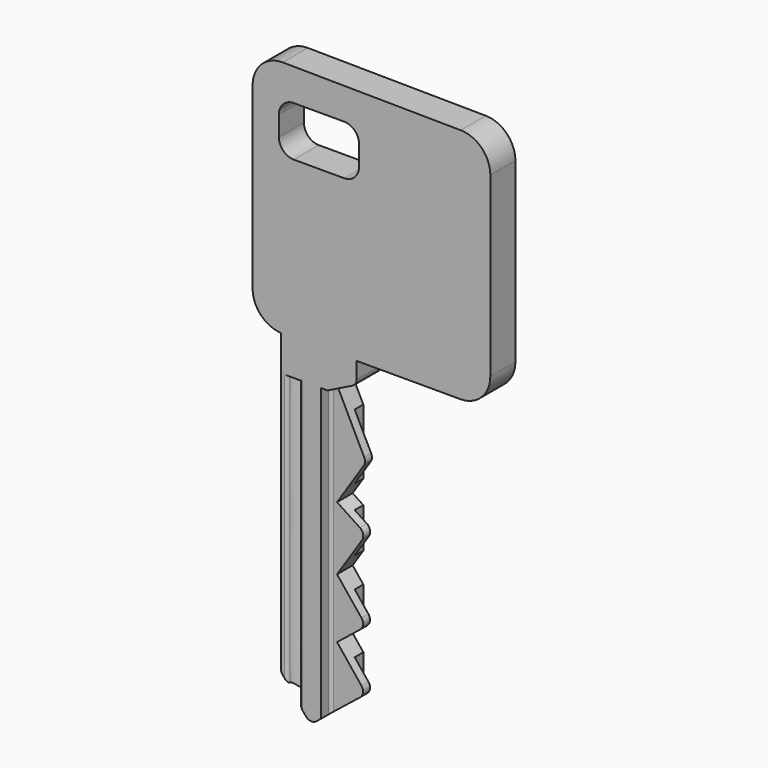
from build123d import *

# Parameters (mm, degrees)
F0_W        = 13.6487651616
F0_H        = 8.4716491401
F1_DEPTH    = 5.334
F2_T1_DEPTH = 30.734
F2_T3_DEPTH = 30.9986733357
F2_T5_DEPTH = 30.6972722749
F2_T7_DEPTH = 30.472056174
F3_R        = 2.54
F4_R        = 1.27
F6_DEPTH    = 52.1462
F7_W        = 6.471471861
F7_H        = 2.0470987074
F8_DEPTH    = 58.928
F9_W        = 3.0602971092
F9_H        = 1.8379887333
F10_DEPTH   = 54.61
F12_DEPTH   = 55.626
F13_R       = 0.508


# Not quite as in the source:
# - a fillet or chamfer that OpenCascade refuses, or shapes differently, is made with other operations: its cross-section is extruded or revolved along the edge and cut away or added


with BuildPart() as f1:
    # F0 (on Front) → F1 (new body)
    with BuildSketch(Plane.XZ):
        Polygon((40.4473207891, 46.2965518236), (0, 46.7158481479), (0, 6.0438592918), (4.8069125041, 6.0438592918), (4.8069125041, -44.6913056076), (9.8384991288, -50.9807877243), (17.7003503195, -44.6913056076), (12.7505768579, -38.5040899258), (17.7003503195, -34.5442704236), (12.7505768579, -28.3570547418), (17.7003503195, -20.7912679762), (12.7505768579, -17.5529719363), (17.7003503195, -9.9871851707), (12.7505768579, 0), (17.7003503195, 2.4531694269), (17.7003503195, 6.0438592918), (40.4473207891, 6.0438592918), align=None)
        with Locations((11.2955300137, 36.9457956403)):
            Rectangle(F0_W, F0_H, mode=Mode.SUBTRACT)
    extrude(amount=F1_DEPTH)

    # F2: fillet of radius 5.08 on 4 edges, made by hand

    # F2_s2 → F2_t1 (cut)
    with BuildSketch(Plane.XZ.offset(-12.7)):
        with BuildLine():
            ThreePointArc((35.3673207891, 6.0438592918), (38.9594232375, 7.5317568434), (40.4473207891, 11.1238592918))
            Line((40.4473207891, 11.1238592918), (40.4473207891, 6.0438592918))
            Line((40.4473207891, 6.0438592918), (35.3673207891, 6.0438592918))
        make_face()
    extrude(amount=F2_T1_DEPTH, mode=Mode.SUBTRACT)

    # F2_s4 → F2_t3 (cut)
    with BuildSketch(Plane.XZ.offset(-12.8323366678)):
        with BuildLine():
            ThreePointArc((5.1326588868, 46.6626405444), (1.5065637787, 45.1935856581), (0, 41.5829134807))
            Line((0, 41.5829134807), (0, 46.7158481479))
            Line((0, 46.7158481479), (5.1326588868, 46.6626405444))
        make_face()
    extrude(amount=F2_T3_DEPTH, mode=Mode.SUBTRACT)

    # F2_s6 → F2_t5 (cut)
    with BuildSketch(Plane.XZ.offset(-12.6816361374)):
        with BuildLine():
            ThreePointArc((0, 11.1165137468), (1.392610376, 7.6222959859), (4.8069125041, 6.0438592918))
            Line((4.8069125041, 6.0438592918), (0, 6.0438592918))
            Line((0, 6.0438592918), (0, 11.1165137468))
        make_face()
    extrude(amount=F2_T5_DEPTH, mode=Mode.SUBTRACT)

    # F2_s8 → F2_t7 (cut)
    with BuildSketch(Plane.XZ.offset(-12.569028087)):
        with BuildLine():
            ThreePointArc((40.4473207891, 41.2689405888), (38.9779929665, 44.8423768101), (35.4199796759, 46.3486676525))
            Line((35.4199796759, 46.3486676525), (40.4473207891, 46.2965518236))
            Line((40.4473207891, 46.2965518236), (40.4473207891, 41.2689405888))
        make_face()
    extrude(amount=F2_T7_DEPTH, mode=Mode.SUBTRACT)

    # F3
    f3_edges = [f1.edges().sort_by_distance(p)[0] for p in [
        (18.119913, -2.667, 41.18162),
        (4.471147, -2.667, 41.18162),
        (4.471147, -2.667, 32.709971),
        (18.119913, -2.667, 32.709971),
    ]]
    fillet(f3_edges, radius=F3_R)

    # F4
    f4_edges = [f1.edges().sort_by_distance(p)[0] for p in [
        (17.70035, -2.667, 2.453169),
        (17.70035, -2.667, -9.987185),
        (17.70035, -2.667, -20.791268),
        (17.70035, -2.667, -34.54427),
        (17.70035, -2.667, -44.691306),
        (9.838499, -2.667, -50.980788),
        (4.806913, -2.667, -44.691306),
    ]]
    fillet(f4_edges, radius=F4_R)

    # F5 (on Top) → F6 (cut)
    with BuildSketch(Plane.XY):
        with BuildLine():
            add(Edge.make_bspline(
                [(5.9925829992, -5.3615476936), (5.9662371728, -5.1413136829), (5.9117415486, -4.685765632), (6.3531394911, -4.0979348233), (6.8182620743, -3.382318142), (7.2587507478, -3.2452825018), (7.6600250696, -4.1522550659), (8.0135536671, -4.7405594262), (8.0147180391, -5.162214979), (8.0152684823, -5.3615476936)],
                knots=[0, 0, 0, 0, 0.1405767765, 0.2907792323, 0.4524560789, 0.5501663785, 0.7152294594, 0.8653780686, 1, 1, 1, 1], degree=3))
            Line((5.9925829992, -5.3615476936), (8.0152684823, -5.3615476936))
        make_face()
    extrude(amount=-F6_DEPTH, mode=Mode.SUBTRACT)

    # F7 (on Top) → F8 (cut)
    with BuildSketch(Plane.XY):
        with Locations((14.903399162, -4.3372439686)):
            Rectangle(F7_W, F7_H)
    extrude(amount=-F8_DEPTH, mode=Mode.SUBTRACT)

    # F9 (on Top) → F10 (cut)
    with BuildSketch(Plane.XY):
        with Locations((16.1025538109, -0.9189943667)):
            Rectangle(F9_W, F9_H)
    extrude(amount=-F10_DEPTH, mode=Mode.SUBTRACT)

    # F11 (on Top) → F12 (cut)
    with BuildSketch(Plane.XY):
        with BuildLine():
            add(Edge.make_bspline(
                [(11.2238610163, 0), (11.2478981656, -0.3069122797), (11.3009665063, -0.984502007), (10.6443157535, -2.3913685017), (9.025430434, -2.589119864), (8.3644189358, -0.856075456), (8.4617577104, -0.2545179476), (8.5029415786, 0)],
                knots=[0, 0, 0, 0, 0.1796332137, 0.3965876516, 0.6003917954, 0.8309264556, 1, 1, 1, 1], degree=3))
            Line((11.2238610163, 0), (8.5029415786, 0))
        make_face()
    extrude(amount=-F12_DEPTH, mode=Mode.SUBTRACT)

    # F13
    f13_edges = [f1.edges().sort_by_distance(p)[0] for p in [
        (8.015188, -5.334, -24.350824),
        (5.989293, -5.334, -23.084641),
        (11.223861, 0, -24.936249),
        (8.502942, 0, -24.655671),
        (11.667663, -3.313695, -24.758728),
    ]]
    fillet(f13_edges, radius=F13_R)


solid = f1.part
